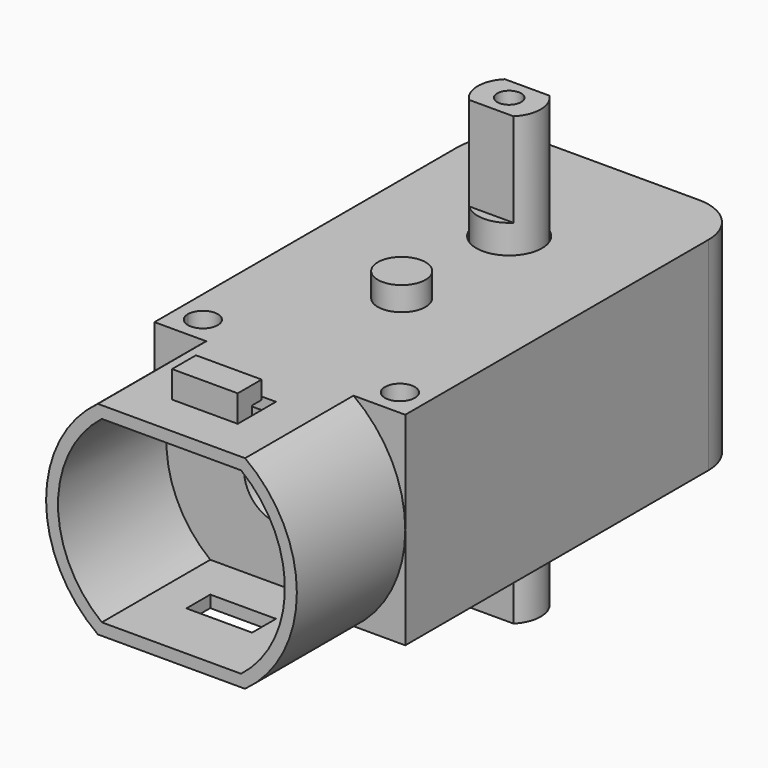
from build123d import *

# Parameters (mm, degrees)
F0_R      = 1.25
F1_DEPTH  = 8.5
F2_R      = 4
F3_T      = -1
F4_W      = 5
F4_H      = 2.8
F5_DEPTH  = 5
F6_R      = 0.125
F7_R      = 1.35
F8_DEPTH  = 2.8
F10_DEPTH = 11.35
F11_R     = 3
F12_DEPTH = 1
F13_R     = 2
F14_DEPTH = 2
F16_DEPTH = 25
F17_W     = 5.5
F17_H     = 1.5
F18_DEPTH = 2.25
F19_W     = 5.5
F19_H     = 1.5
F20_DEPTH = 2.5
F21_W     = 5.5
F21_H     = 1.5
F22_DEPTH = 2.25
F23_W     = 5.5
F23_H     = 1.5
F24_DEPTH = 1
F25_R     = 2.64078
F26_DEPTH = 18.7
F27_R     = 1
F28_DEPTH = 7.85


with BuildPart() as f1:
    # F0 (on Top) → F1 (new body, symmetric)
    with BuildSketch(Plane.XY):
        with BuildLine():
            Line((-8.25, -17.875), (0, -17.875))
            Line((0, -17.875), (0, -7.125))
            ThreePointArc((0, -7.125), (-2, -5.125), (0, -3.125))
            Line((0, -3.125), (0, 3.375))
            ThreePointArc((0, 3.375), (-2.75, 6.125), (0, 8.875))
            Line((0, 8.875), (0, 17.875))
            Line((0, 17.875), (-10.5, 17.875))
            Line((-10.5, 17.875), (-10.5, -15.625))
            Line((-10.5, -15.625), (-9.5, -15.625))
            ThreePointArc((-9.5, -15.625), (-8.25, -14.375), (-7, -15.625))
            ThreePointArc((-7, -15.625), (-7.366117, -16.508883), (-8.25, -16.875))
            Line((-8.25, -16.875), (-8.25, -17.875))
        make_face()
        with BuildLine():
            Line((0, -17.875), (10.5, -17.875))
            Line((10.5, -17.875), (10.5, 17.875))
            Line((10.5, 17.875), (0, 17.875))
            Line((0, 17.875), (0, 8.875))
            ThreePointArc((0, 8.875), (1.944544, 8.069544), (2.75, 6.125))
            ThreePointArc((2.75, 6.125), (1.944544, 4.180456), (0, 3.375))
            Line((0, 3.375), (0, -3.125))
            ThreePointArc((0, -3.125), (1.414214, -3.710786), (2, -5.125))
            ThreePointArc((2, -5.125), (1.414214, -6.539214), (0, -7.125))
            Line((0, -7.125), (0, -17.875))
        make_face()
        with Locations((8.25, -15.625)):
            Circle(F0_R, mode=Mode.SUBTRACT)
        with BuildLine():
            Line((-10.5, -17.875), (-8.25, -17.875))
            Line((-8.25, -17.875), (-8.25, -16.875))
            ThreePointArc((-8.25, -16.875), (-9.133883, -16.508883), (-9.5, -15.625))
            Line((-9.5, -15.625), (-10.5, -15.625))
            Line((-10.5, -15.625), (-10.5, -17.875))
        make_face()
        with BuildLine():
            ThreePointArc((0, -3.125), (-2, -5.125), (0, -7.125))
            ThreePointArc((0, -7.125), (1.414214, -6.539214), (2, -5.125))
            ThreePointArc((2, -5.125), (1.414214, -3.710786), (0, -3.125))
        make_face()
    extrude(amount=F1_DEPTH, both=True)

    # F2
    f2_edges = [f1.edges().sort_by_distance(p)[0] for p in [
        (-10.5, 17.875, 0),
        (10.5, 17.875, 0),
    ]]
    fillet(f2_edges, radius=F2_R)

    # F3 (hollow: no face is removed)
    offset(amount=F3_T, mode=Mode.SUBTRACT)

    # F4 (on face) → F5 (join)
    with BuildSketch(Plane(origin=(0, 17.875, 0), x_dir=(-1, 0, 0), z_dir=(0, 1, 0))):
        Rectangle(F4_W, F4_H)
    extrude(amount=F5_DEPTH)

    # F6
    f6_edges = [f1.edges().sort_by_distance(p)[0] for p in [
        (-2.5, 22.875, 0),
        (2.5, 22.875, 0),
        (2.5, 17.875, 0),
        (-2.5, 17.875, 0),
    ]]
    fillet(f6_edges, radius=F6_R)

    # F7 (on face) → F8 (cut)
    with BuildSketch(Plane.XY.offset(1.4)):
        with Locations((0, 20.375)):
            Circle(F7_R)
    extrude(amount=-F8_DEPTH, mode=Mode.SUBTRACT)

    # F9 (on face) → F10 (join)
    with BuildSketch(Plane.XZ.offset(17.875)):
        with BuildLine():
            Line((-4.242641, 8.5), (-6.164414, 8.5))
            ThreePointArc((-6.164414, 8.5), (-10.5, 0), (-6.164414, -8.5))
            Line((-6.164414, -8.5), (-4.242641, -8.5))
            ThreePointArc((-4.242641, -8.5), (-5.061553, -8.039321), (-5.830952, -7.5))
            ThreePointArc((-5.830952, -7.5), (-9.5, 0), (-5.830952, 7.5))
            ThreePointArc((-5.830952, 7.5), (-5.061553, 8.039321), (-4.242641, 8.5))
        make_face()
        with BuildLine():
            Line((-2.465676, 8.5), (-4.242641, 8.5))
            ThreePointArc((-4.242641, 8.5), (-5.061553, 8.039321), (-5.830952, 7.5))
            Line((-5.830952, 7.5), (-2.465676, 7.5))
            Line((-2.465676, 7.5), (-2.465676, 8.5))
        make_face()
        with BuildLine():
            ThreePointArc((-5.830952, -7.5), (-5.061553, -8.039321), (-4.242641, -8.5))
            Line((-4.242641, -8.5), (-1.975537, -8.5))
            Line((-1.975537, -8.5), (-1.975537, -7.5))
            Line((-1.975537, -7.5), (-5.830952, -7.5))
        make_face()
        with BuildLine():
            Line((4.242641, 8.5), (-2.465676, 8.5))
            Line((-2.465676, 8.5), (-2.465676, 7.5))
            Line((-2.465676, 7.5), (5.830952, 7.5))
            ThreePointArc((5.830952, 7.5), (5.061553, 8.039321), (4.242641, 8.5))
        make_face()
        with BuildLine():
            Line((-1.975537, -7.5), (-1.975537, -8.5))
            Line((-1.975537, -8.5), (4.242641, -8.5))
            ThreePointArc((4.242641, -8.5), (5.061553, -8.039321), (5.830952, -7.5))
            Line((5.830952, -7.5), (-1.975537, -7.5))
        make_face()
        with BuildLine():
            Line((6.164414, 8.5), (4.242641, 8.5))
            ThreePointArc((4.242641, 8.5), (5.061553, 8.039321), (5.830952, 7.5))
            ThreePointArc((5.830952, 7.5), (9.5, 0), (5.830952, -7.5))
            ThreePointArc((5.830952, -7.5), (5.061553, -8.039321), (4.242641, -8.5))
            Line((4.242641, -8.5), (6.164414, -8.5))
            ThreePointArc((6.164414, -8.5), (10.5, 0), (6.164414, 8.5))
        make_face()
    extrude(amount=F10_DEPTH)

    # F11 (on face) → F12 (cut)
    with BuildSketch(Plane.XZ.offset(17.875)):
        Circle(F11_R)
    extrude(amount=-F12_DEPTH, mode=Mode.SUBTRACT)

    # F13 (on face) → F14 (join)
    with BuildSketch(Plane.XY.offset(8.5)):
        with Locations((0, -5.125)):
            Circle(F13_R)
    extrude(amount=F14_DEPTH)

    # F15 (on face) → F16 (cut)
    with BuildSketch(Plane.XY.offset(8.5)):
        Polygon((-1.504724, -24.225), (2.75, -24.225), (2.75, -21.725), (-2.75, -21.725), (-2.75, -24.225), align=None)
    extrude(amount=-F16_DEPTH, mode=Mode.SUBTRACT)

    # F17 (on face) → F18 (join)
    with BuildSketch(Plane.XY.offset(8.5)):
        with Locations((0, -24.975)):
            Rectangle(F17_W, F17_H)
    extrude(amount=F18_DEPTH)

    # F19 (on face) → F20 (join)
    with BuildSketch(Plane.XZ.offset(25.725)):
        with Locations((0, 10)):
            Rectangle(F19_W, F19_H)
    extrude(amount=-F20_DEPTH)

    # F21 (on face) → F22 (join)
    with BuildSketch(Plane(origin=(0, 0, -8.5), x_dir=(1, 0, 0), z_dir=(0, 0, -1))):
        with Locations((0, 24.975)):
            Rectangle(F21_W, F21_H)
    extrude(amount=F22_DEPTH)

    # F23 (on face) → F24 (join)
    with BuildSketch(Plane(origin=(0, -24.225, 0), x_dir=(-1, 0, 0), z_dir=(0, 1, 0))):
        with Locations((0, -10)):
            Rectangle(F23_W, F23_H)
    extrude(amount=F24_DEPTH)


with BuildPart() as f26:
    # F25 (on face) → F26 (new body)
    with BuildSketch(Plane.XY):
        with Locations((0, 6.125)):
            Circle(F25_R)
    extrude(amount=F26_DEPTH)

    # F27 (on face) → F28 (cut)
    with BuildSketch(Plane.XY.offset(18.7)):
        with BuildLine():
            Line((1.859595, 4.25), (-1.859595, 4.25))
            ThreePointArc((-1.859595, 4.25), (0, 3.48422), (1.859595, 4.25))
        make_face()
        with BuildLine():
            ThreePointArc((1.859595, 8), (0, 8.76578), (-1.859595, 8))
            Line((-1.859595, 8), (1.859595, 8))
        make_face()
        with Locations((0, 6.125)):
            Circle(F27_R)
    extrude(amount=-F28_DEPTH, mode=Mode.SUBTRACT)

    # F29: F26 across plane


with BuildPart() as f26_1:
    add(f26.part)
    add(f26.part.mirror(Plane.XY))


solid = Compound([f1.part, f26_1.part])
